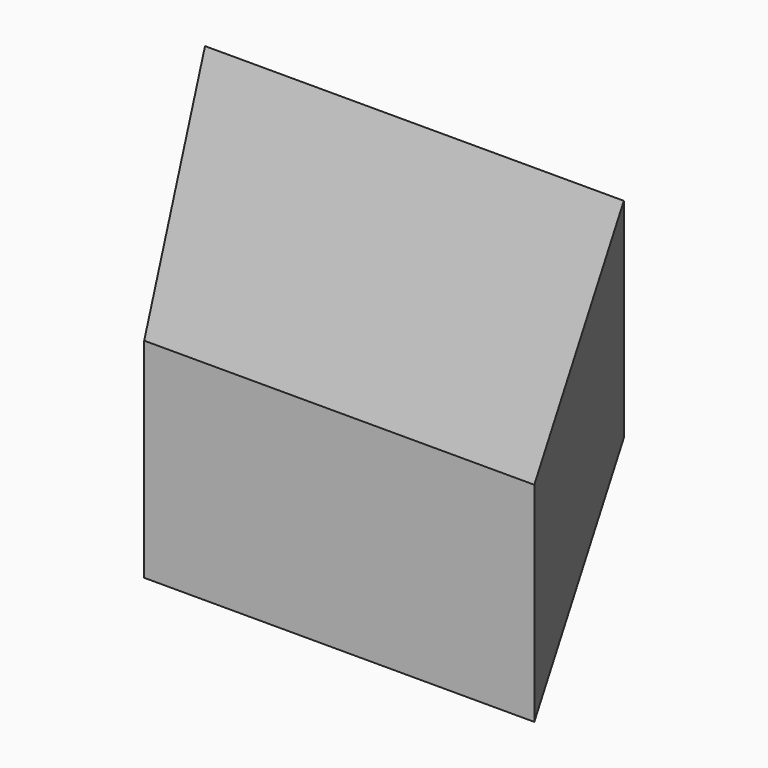
from build123d import *

# Parameters (mm, degrees)
F1_DEPTH = 25.4


# Not quite as in the source:
# - ends of sketch curves that miss each other by under 0.0002 mm in the source are joined


with BuildPart() as f1:
    # F0 (on Top) → F1 (new body)
    with BuildSketch(Plane.XY):
        Polygon((-33.3464348924, 50.9338825941), (-3.0268e-06, 7.4506e-06), (47.4594160914, 0), (17.6039151847, 50.9338825941), align=None)
    extrude(amount=F1_DEPTH)


solid = f1.part
